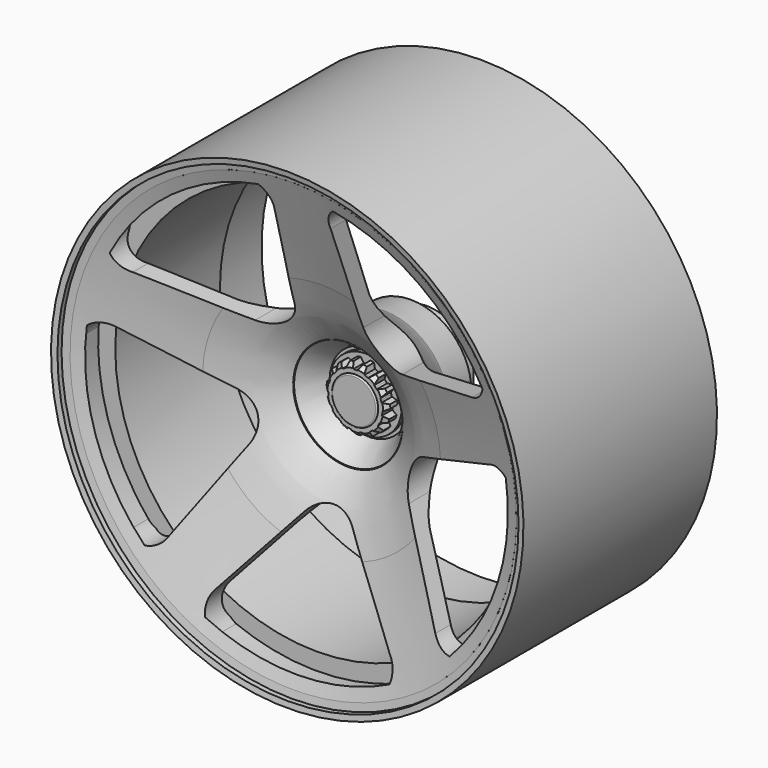
from build123d import *

# Parameters (mm, degrees)
F3_DEPTH  = 79.9052135477
F5_R      = 16.2841993911
F6_DEPTH  = 25
F7_R      = 12.5
F8_DEPTH  = 1.5
F10_DEPTH = 6
F13_R     = 7.9523329074
F14_DEPTH = 0.5
F15_R     = 0.49999
F16_R     = 79.6764965697
F16_R_2   = 69.9009802276
F17_DEPTH = 22.7
F18_R     = 19
F19_DEPTH = 22.5


# Not quite as in the source:
# - a fillet or chamfer is up to 0.001 mm smaller than in the source, because OpenCascade refuses the exact size


with BuildPart() as f1:
    # F0 (on Right) → F1 (revolve)
    with BuildSketch(Plane.YZ):
        with BuildLine():
            Line((-1.373420301, 77.4389281869), (-1.3914429583, 77.4389281869))
            Line((-1.3914429583, 77.4389281869), (10.8794942498, 41.2581264973))
            add(Edge.make_bspline(
                [(10.8794942498, 41.2581264973), (18.0547758937, 20.7232777029), (23.3377031982, 16.0578545183), (31.9949798286, 13.4048163891)],
                knots=[0, 0, 0, 0, 34.9524049989, 34.9524049989, 34.9524049989, 34.9524049989], degree=3))
            Line((31.9949798286, 13.4048163891), (31.9949798286, 0))
            Line((31.9949798286, 0), (49.5772249997, 0))
            Line((49.5772249997, 0), (49.5772249997, 20.9933258593))
            Line((49.5772249997, 20.9933258593), (38.1912440062, 22.2220420837))
            add(Edge.make_bspline(
                [(38.1912440062, 22.2220420837), (33.309340477, 23.849343881), (19.0382879227, 34.485783428), (16.9671755284, 42.0305468142)],
                knots=[0, 0, 0, 0, 29.0316713677, 29.0316713677, 29.0316713677, 29.0316713677], degree=3))
            Line((16.9671755284, 42.0305468142), (8.8946735486, 66.8536573648))
            add(Edge.make_bspline(
                [(8.8946735486, 66.8536573648), (5.8300439268, 75.6170749664), (9.7822928801, 76.194010675), (12.1492771432, 76.0460719466)],
                knots=[0, 0, 0, 0, 9.7515604085, 9.7515604085, 9.7515604085, 9.7515604085], degree=3))
            Line((12.1492771432, 76.0460719466), (79.9042135477, 76.0460719466))
            Line((79.9042135477, 76.0460719466), (79.9042135477, 81.9431841373))
            Line((79.9042135477, 81.9431841373), (-4.0100626432, 81.9431841373))
            Line((-4.0100626432, 81.9431841373), (-3.6750880512, 79.9715518951))
            Line((-3.6750880512, 79.9715518951), (-1.8980908117, 79.9715518951))
            Line((-1.8980908117, 79.9715518951), (-1.373420301, 77.4389281869))
        make_face()
    revolve(axis=Axis((0, 6.5627768636, 0), (0, 1, 0)))

    # F2 (on Front) → F3 (cut, through all)
    with BuildSketch(Plane.XZ):
        with BuildLine():
            Line((-11.9682861573, 30.7326176724), (-9.751479551, 64.9884316832))
            ThreePointArc((-9.751479551, 64.9884316832), (-12.288415463, 71.3748405533), (-18.8385986029, 73.4526670407))
            ThreePointArc((-18.8385986029, 73.4526670407), (-44.5717486769, 61.3477490426), (-64.0361905098, 40.6146943569))
            ThreePointArc((-64.0361905098, 40.6146943569), (-64.4939701233, 33.5522102634), (-58.7942985346, 29.3567379984))
            Line((-58.7942985346, 29.3567379984), (-25.530052484, 20.8794176812))
            ThreePointArc((-25.530052484, 20.8794176812), (-16.436274739, 22.6225913906), (-11.9682861573, 30.7326176724))
        make_face()
        with BuildLine():
            Line((25.530052484, 20.8794176812), (58.7942985346, 29.3567379984))
            ThreePointArc((58.7942985346, 29.3567379984), (64.0841779958, 33.7430163028), (64.0361905098, 40.6146943569))
            ThreePointArc((64.0361905098, 40.6146943569), (44.5717486769, 61.3477490426), (18.8385986029, 73.4526670407))
            ThreePointArc((18.8385986029, 73.4526670407), (11.9803154043, 71.7056137177), (9.751479551, 64.9884316832))
            Line((9.751479551, 64.9884316832), (11.9682861573, 30.7326176724))
            ThreePointArc((11.9682861573, 30.7326176724), (16.436274739, 22.6225913906), (25.530052484, 20.8794176812))
        make_face()
        with BuildLine():
            Line((27.746726327, -17.8284278801), (46.0883543901, -46.8449698014))
            ThreePointArc((46.0883543901, -46.8449698014), (51.8946156055, -50.5205095952), (58.415140848, -48.3514054854))
            ThreePointArc((58.415140848, -48.3514054854), (72.1186042972, -23.432755001), (75.6790847468, 4.7815504386))
            ThreePointArc((75.6790847468, 4.7815504386), (71.8982122391, 10.7642961983), (64.8210443377, 10.8083216574))
            Line((64.8210443377, 10.8083216574), (32.9268601163, -1.8856153964))
            ThreePointArc((32.9268601163, -1.8856153964), (26.5944511761, -8.6410609976), (27.746726327, -17.8284278801))
        make_face()
        with BuildLine():
            Line((-8.3816325373, -31.8979920771), (-30.310129036, -58.3085215376))
            ThreePointArc((-30.310129036, -58.3085215376), (-32.0115417185, -64.9664083617), (-27.9336480081, -70.4975063507))
            ThreePointArc((-27.9336480081, -70.4975063507), (0, -75.8299880833), (27.9336480081, -70.4975063507))
            ThreePointArc((27.9336480081, -70.4975063507), (32.4552234898, -65.0529128022), (30.310129036, -58.3085215376))
            Line((30.310129036, -58.3085215376), (8.3816325373, -31.8979920771))
            ThreePointArc((8.3816325373, -31.8979920771), (0, -27.963060786), (-8.3816325373, -31.8979920771))
        make_face()
        with BuildLine():
            Line((-32.9268601163, -1.8856153964), (-64.8210443377, 10.8083216574))
            ThreePointArc((-64.8210443377, 10.8083216574), (-71.6788364198, 10.3690611007), (-75.6790847468, 4.7815504386))
            ThreePointArc((-75.6790847468, 4.7815504386), (-72.1186042972, -23.432755001), (-58.415140848, -48.3514054854))
            ThreePointArc((-58.415140848, -48.3514054854), (-51.8397810099, -50.9692073773), (-46.0883543901, -46.8449698014))
            Line((-46.0883543901, -46.8449698014), (-27.746726327, -17.8284278801))
            ThreePointArc((-27.746726327, -17.8284278801), (-26.5944511761, -8.6410609976), (-32.9268601163, -1.8856153964))
        make_face()
    extrude(amount=-F3_DEPTH, mode=Mode.SUBTRACT)

    # F18 (on Front) → F19 (cut)
    with BuildSketch(Plane.XZ):
        Circle(F18_R)
    extrude(amount=-F19_DEPTH, mode=Mode.SUBTRACT)


with BuildPart() as f6:
    # F5 (on offset) → F6 (new body)
    with BuildSketch(Plane.XZ.offset(-31.5)):
        Circle(F5_R)
    extrude(amount=-F6_DEPTH)


with BuildPart() as f8:
    # F7 (on offset) → F8 (new body)
    with BuildSketch(Plane.XZ.offset(-31.5)):
        Circle(F7_R)
    extrude(amount=F8_DEPTH)


with BuildPart() as f10:
    # F9 (on offset) → F10 (new body)
    with BuildSketch(Plane.XZ.offset(-31.5)):
        with BuildLine():
            ThreePointArc((-1.9532975735, -9.1895425773), (-1.634477598, -9.2515699842), (-1.313704066, -9.3025397509))
            Line((-1.313704066, -9.3025397509), (-0.6322512054, -11.0529381782))
            ThreePointArc((-0.6322512054, -11.0529381782), (0, -11.0710064564), (0.6322512054, -11.0529381782))
            Line((0.6322512054, -11.0529381782), (1.313704066, -9.3025397509))
            ThreePointArc((1.313704066, -9.3025397509), (1.634477598, -9.2515699842), (1.9532975735, -9.1895425773))
            ThreePointArc((1.9532975735, -9.1895425773), (2.2697829332, -9.1165316665), (2.5835554082, -9.0326245158))
            Line((2.5835554082, -9.0326245158), (3.9180447539, -10.3545211991))
            ThreePointArc((3.9180447539, -10.3545211991), (4.5029840015, -10.1138676598), (5.0732251875, -9.8402017334))
            Line((5.0732251875, -9.8402017334), (4.9838121725, -7.9639613522))
            ThreePointArc((4.9838121725, -7.9639613522), (5.2561221039, -7.7869278037), (5.522149825, -7.6005871813))
            ThreePointArc((5.522149825, -7.6005871813), (5.781577375, -7.4051622026), (6.0340946815, -7.2008864431))
            Line((6.0340946815, -7.2008864431), (7.790875181, -7.8657134369))
            ThreePointArc((7.790875181, -7.8657134369), (8.2273611609, -7.4079492632), (8.6369924459, -6.9260050135))
            Line((8.6369924459, -6.9260050135), (7.7921738779, -5.2483416854))
            ThreePointArc((7.7921738779, -5.2483416854), (7.9689353475, -4.9758550639), (8.1361722046, -4.6974212125))
            ThreePointArc((8.1361722046, -4.6974212125), (8.2936845647, -4.4133729201), (8.4412841663, -4.1240496863))
            Line((8.4412841663, -4.1240496863), (10.3165925114, -4.0168523637))
            ThreePointArc((10.3165925114, -4.0168523637), (10.5291528323, -3.4211291399), (10.7073452457, -2.814239106))
            Line((10.7073452457, -2.814239106), (9.2531979302, -1.6252360615))
            ThreePointArc((9.2531979302, -1.6252360615), (9.3038472741, -1.3044117794), (9.3433764952, -0.9820284413))
            ThreePointArc((9.3433764952, -0.9820284413), (9.3717383474, -0.6584713655), (9.388898932, -0.334127273))
            Line((9.388898932, -0.334127273), (11.0584772733, 0.5265589752))
            ThreePointArc((11.0584772733, 0.5265589752), (11.0103583246, 1.1572352917), (10.9263007795, 1.7841343095))
            Line((10.9263007795, 1.7841343095), (9.1142599976, 2.2788876423))
            ThreePointArc((9.1142599976, 2.2788876423), (9.0300394842, 2.592576152), (8.9350261079, 2.9031659688))
            ThreePointArc((8.9350261079, 2.9031659688), (8.8293334302, 3.2102858703), (8.713087777, 3.5135687813))
            Line((8.713087777, 3.5135687813), (9.8882508515, 4.9789234837))
            ThreePointArc((9.8882508515, 4.9789234837), (9.5877728367, 5.5355032282), (9.2559996461, 6.0740146945))
            Line((9.2559996461, 6.0740146945), (7.399383711, 5.7889709697))
            ThreePointArc((7.399383711, 5.7889709697), (7.1948558322, 6.0412841139), (6.9817285343, 6.2863766085))
            ThreePointArc((6.9817285343, 6.2863766085), (6.760256551, 6.5239555145), (6.5307045894, 6.7537368735))
            Line((6.5307045894, 6.7537368735), (7.0082560255, 8.5703868897))
            ThreePointArc((7.0082560255, 8.5703868897), (6.5073743231, 8.9566323681), (5.9852520858, 9.3136427582))
            Line((5.9852520858, 9.3136427582), (4.4050867595, 8.2980886252))
            ThreePointArc((4.4050867595, 8.2980886252), (4.1156162435, 8.4453991692), (3.8212266702, 8.5826156226))
            ThreePointArc((3.8212266702, 8.5826156226), (3.5222698991, 8.709573982), (3.2191032487, 8.8261225045))
            Line((3.2191032487, 8.8261225045), (2.9164700647, 10.6799525429))
            ThreePointArc((2.9164700647, 10.6799525429), (2.3017916714, 10.829078403), (1.6796000655, 10.9428573772))
            Line((1.6796000655, 10.9428573772), (0.6491102883, 9.3723913717))
            ThreePointArc((0.6491102883, 9.3723913717), (0.3247492172, 9.3892279841), (0, 9.394842425))
            ThreePointArc((0, 9.394842425), (-0.3247492172, 9.3892279841), (-0.6491102883, 9.3723913717))
            Line((-0.6491102883, 9.3723913717), (-1.6796000655, 10.9428573772))
            ThreePointArc((-1.6796000655, 10.9428573772), (-2.3017916714, 10.829078403), (-2.9164700647, 10.6799525429))
            Line((-2.9164700647, 10.6799525429), (-3.2191032487, 8.8261225045))
            ThreePointArc((-3.2191032487, 8.8261225045), (-3.5222698991, 8.709573982), (-3.8212266702, 8.5826156226))
            ThreePointArc((-3.8212266702, 8.5826156226), (-4.1156162435, 8.4453991692), (-4.4050867595, 8.2980886252))
            Line((-4.4050867595, 8.2980886252), (-5.9852520858, 9.3136427582))
            ThreePointArc((-5.9852520858, 9.3136427582), (-6.5073743231, 8.9566323681), (-7.0082560255, 8.5703868897))
            Line((-7.0082560255, 8.5703868897), (-6.5307045894, 6.7537368735))
            ThreePointArc((-6.5307045894, 6.7537368735), (-6.760256551, 6.5239555145), (-6.9817285343, 6.2863766085))
            ThreePointArc((-6.9817285343, 6.2863766085), (-7.1948558322, 6.0412841139), (-7.399383711, 5.7889709697))
            Line((-7.399383711, 5.7889709697), (-9.2559996461, 6.0740146945))
            ThreePointArc((-9.2559996461, 6.0740146945), (-9.5877728367, 5.5355032282), (-9.8882508515, 4.9789234837))
            Line((-9.8882508515, 4.9789234837), (-8.713087777, 3.5135687813))
            ThreePointArc((-8.713087777, 3.5135687813), (-8.8293334302, 3.2102858703), (-8.9350261079, 2.9031659688))
            ThreePointArc((-8.9350261079, 2.9031659688), (-9.0300394842, 2.592576152), (-9.1142599976, 2.2788876423))
            Line((-9.1142599976, 2.2788876423), (-10.9263007795, 1.7841343095))
            ThreePointArc((-10.9263007795, 1.7841343095), (-11.0103583246, 1.1572352917), (-11.0584772733, 0.5265589752))
            Line((-11.0584772733, 0.5265589752), (-9.388898932, -0.334127273))
            ThreePointArc((-9.388898932, -0.334127273), (-9.3717383474, -0.6584713655), (-9.3433764952, -0.9820284413))
            ThreePointArc((-9.3433764952, -0.9820284413), (-9.3038472741, -1.3044117794), (-9.2531979302, -1.6252360615))
            Line((-9.2531979302, -1.6252360615), (-10.7073452457, -2.814239106))
            ThreePointArc((-10.7073452457, -2.814239106), (-10.5291528323, -3.4211291399), (-10.3165925114, -4.0168523637))
            Line((-10.3165925114, -4.0168523637), (-8.4412841663, -4.1240496863))
            ThreePointArc((-8.4412841663, -4.1240496863), (-8.2936845647, -4.4133729201), (-8.1361722046, -4.6974212125))
            ThreePointArc((-8.1361722046, -4.6974212125), (-7.9689353475, -4.9758550639), (-7.7921738779, -5.2483416854))
            Line((-7.7921738779, -5.2483416854), (-8.6369924459, -6.9260050135))
            ThreePointArc((-8.6369924459, -6.9260050135), (-8.2273611609, -7.4079492632), (-7.790875181, -7.8657134369))
            Line((-7.790875181, -7.8657134369), (-6.0340946815, -7.2008864431))
            ThreePointArc((-6.0340946815, -7.2008864431), (-5.781577375, -7.4051622026), (-5.522149825, -7.6005871813))
            ThreePointArc((-5.522149825, -7.6005871813), (-5.2561221039, -7.7869278037), (-4.9838121725, -7.9639613522))
            Line((-4.9838121725, -7.9639613522), (-5.0732251875, -9.8402017334))
            ThreePointArc((-5.0732251875, -9.8402017334), (-4.5029840015, -10.1138676598), (-3.9180447539, -10.3545211991))
            Line((-3.9180447539, -10.3545211991), (-2.5835554082, -9.0326245158))
            ThreePointArc((-2.5835554082, -9.0326245158), (-2.2697829332, -9.1165316665), (-1.9532975735, -9.1895425773))
        make_face()
    extrude(amount=F10_DEPTH)

    # F11 (on Right) → F12 (revolve, cut)
    with BuildSketch(Plane.YZ):
        Polygon((17.0979294926, 0.9799834806), (27.729421854, 11.9285192341), (28.4050200135, 17.950873822), (17.0979294926, 17.950873822), align=None)
    revolve(axis=Axis((0, 19.0811585635, 0), (0, 1, 0)), mode=Mode.SUBTRACT)


with BuildPart() as f14:
    # F13 (on face) → F14 (new body)
    with BuildSketch(Plane.XZ.offset(-25.5)):
        Circle(F13_R)
    extrude(amount=F14_DEPTH)

    # F15 (radius 0.5 in the source; OpenCascade refuses exactly that, so slightly less here)
    f15_edges = [f14.edges().sort_by_distance(p)[0] for p in [
        (-7.952333, 25, 0),
    ]]
    fillet(f15_edges, radius=F15_R)


with BuildPart() as f17:
    # F16 (on offset) → F17 (new body, symmetric)
    with BuildSketch(Plane.XZ.offset(-31.5)):
        Circle(F16_R)
        Circle(F16_R_2, mode=Mode.SUBTRACT)
    extrude(amount=F17_DEPTH, both=True)


solid = Compound([f1.part, f6.part, f8.part, f10.part, f14.part, f17.part])
